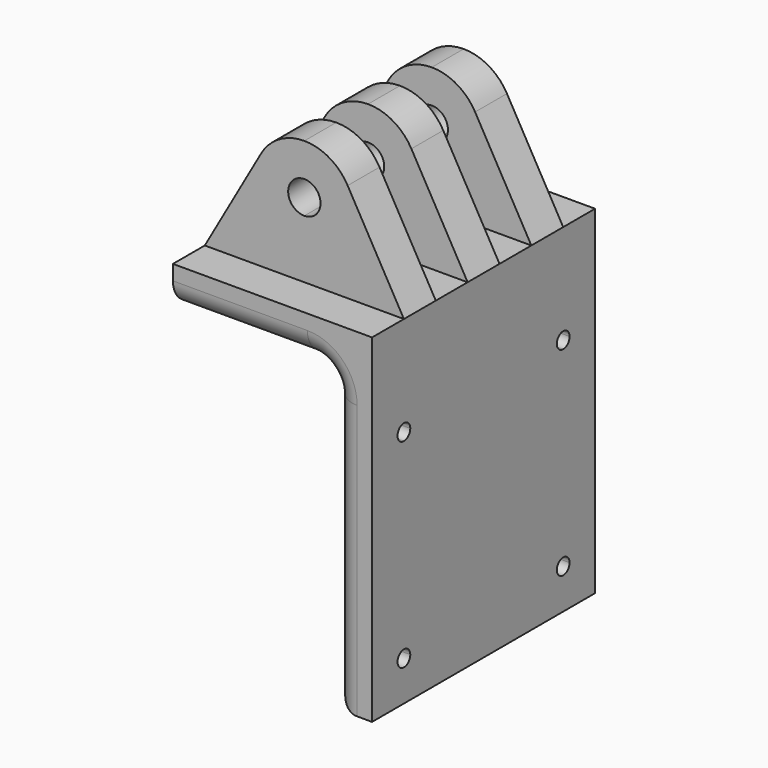
from build123d import *

# Parameters (mm, degrees)
F1_DEPTH      = 40
F2_W          = 8
F2_H          = 25
F3_DEPTH      = 40
F5_DEPTH      = 48
F5_DEPTH_BACK = 8
F6_R          = 5
F8_DEPTH      = 25


with BuildPart() as f1:
    # F0 (on Front) → F1 (new body)
    with BuildSketch(Plane.XZ):
        with BuildLine():
            ThreePointArc((20, 25), (14.9661749692, 23.6406368723), (11.3009091661, 19.9321211119))
            ThreePointArc((11.3009091661, 19.9321211119), (11.3593631277, 9.9661749692), (20, 5))
            ThreePointArc((20, 5), (27.0710678119, 7.9289321881), (30, 15))
            ThreePointArc((30, 15), (29.6693047408, 17.5504011116), (28.6990908339, 19.9321211119))
            ThreePointArc((28.6990908339, 19.9321211119), (25.0338250308, 23.6406368723), (20, 25))
        make_face()
        with BuildLine():
            ThreePointArc((23.25, 15), (22.2980970389, 12.7019029611), (20, 11.75))
            ThreePointArc((20, 11.75), (17.7019029611, 17.2980970389), (23.25, 15))
        make_face(mode=Mode.SUBTRACT)
        with BuildLine():
            Line((11.3009091661, 19.9321211119), (0, 0))
            Line((0, 0), (20, 0))
            Line((20, 0), (20, 5))
            ThreePointArc((20, 5), (11.3593631277, 9.9661749692), (11.3009091661, 19.9321211119))
        make_face()
        with BuildLine():
            Line((20, 5), (20, 0))
            Line((20, 0), (40, 0))
            Line((40, 0), (28.6990908339, 19.9321211119))
            ThreePointArc((28.6990908339, 19.9321211119), (29.6693047408, 17.5504011116), (30, 15))
            ThreePointArc((30, 15), (27.0710678119, 7.9289321881), (20, 5))
        make_face()
    extrude(amount=F1_DEPTH)

    # F2 (on Right) → F3 (cut)
    with BuildSketch(Plane.YZ):
        with Locations((-28, 12.5)):
            Rectangle(F2_W, F2_H)
        with Locations((-12, 12.5)):
            Rectangle(F2_W, F2_H)
    extrude(amount=F3_DEPTH, mode=Mode.SUBTRACT)


with BuildPart() as f5:
    # F4 (on face) → F5 (new body, two sides)
    with BuildSketch(Plane.XZ.offset(40)) as f5_sk:
        Polygon((40, 0), (0, 0), (0, -8), (32, -8), (32, -68), (40, -68), align=None)
    extrude(amount=-F5_DEPTH)
    extrude(f5_sk.sketch, amount=F5_DEPTH_BACK)

    # F6
    f6_edges = [f5.edges().sort_by_distance(p)[0] for p in [
        (32, -48, -38),
        (16, -48, -8),
        (32, -20, -68),
        (32, -20, -8),
        (32, 8, -38),
        (16, 8, -8),
    ]]
    fillet(f6_edges, radius=F6_R)

    # F7 (on face) → F8 (cut)
    with BuildSketch(Plane.YZ.offset(40)):
        with BuildLine():
            ThreePointArc((-1.6, -20), (-1.1313708499, -21.1313708499), (0, -21.6))
            Line((0, -21.6), (0, -20))
            Line((0, -20), (-1.6, -20))
        make_face()
        with BuildLine():
            Line((0, -20), (0, -21.6))
            ThreePointArc((0, -21.6), (1.1313708499, -21.1313708499), (1.6, -20))
            ThreePointArc((1.6, -20), (0, -18.4), (-1.6, -20))
            Line((-1.6, -20), (0, -20))
        make_face()
        with BuildLine():
            ThreePointArc((-38.4, -20), (-41.1313708499, -18.8686291501), (-40, -21.6))
            Line((-40, -21.6), (-40, -20))
            Line((-40, -20), (-38.4, -20))
        make_face()
        with BuildLine():
            Line((-40, -20), (-40, -21.6))
            ThreePointArc((-40, -21.6), (-38.8686291501, -21.1313708499), (-38.4, -20))
            Line((-38.4, -20), (-40, -20))
        make_face()
        with BuildLine():
            ThreePointArc((0, -58.4), (-1.1313708499, -58.8686291501), (-1.6, -60))
            Line((-1.6, -60), (0, -60))
            Line((0, -60), (0, -58.4))
        make_face()
        with BuildLine():
            Line((0, -60), (-1.6, -60))
            ThreePointArc((-1.6, -60), (0, -61.6), (1.6, -60))
            ThreePointArc((1.6, -60), (1.1313708499, -58.8686291501), (0, -58.4))
            Line((0, -58.4), (0, -60))
        make_face()
        with BuildLine():
            Line((-40, -60), (-38.4, -60))
            ThreePointArc((-38.4, -60), (-38.8686291501, -58.8686291501), (-40, -58.4))
            Line((-40, -58.4), (-40, -60))
        make_face()
        with BuildLine():
            ThreePointArc((-40, -58.4), (-41.1313708499, -61.1313708499), (-38.4, -60))
            Line((-38.4, -60), (-40, -60))
            Line((-40, -60), (-40, -58.4))
        make_face()
    extrude(amount=-F8_DEPTH, mode=Mode.SUBTRACT)


solid = Compound([f1.part, f5.part])
